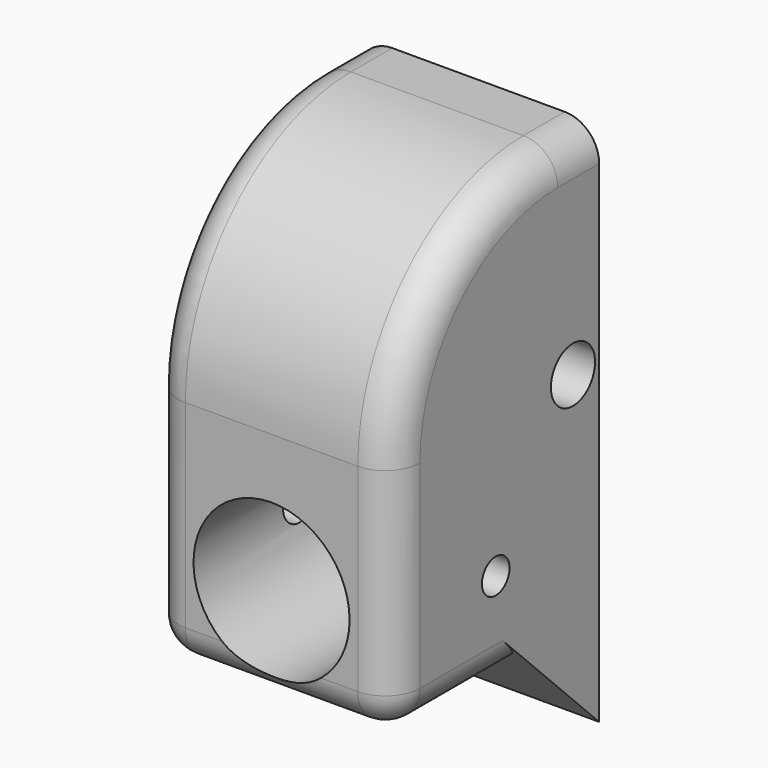
from build123d import *

# Parameters (mm, degrees)
F0_W         = 14
F0_H         = 30.5
F0_R         = 4.525
F1_DEPTH     = 15
F3_DEPTH     = 14.001
F4_R         = 1.6
F4_R_2       = 1
F5_DEPTH     = 14.001
F6_R         = 12
F7_T1_DEPTH  = 10
F7_T3_DEPTH  = 11.5
F7_T5_DEPTH  = 8
F7_S9_W      = 2
F7_S9_H      = 2
F7_T10_DEPTH = 2
F7_S15_W     = 2
F7_S15_H     = 2
F7_T16_DEPTH = 2
F7_T22_DEPTH = 13
F7_T25_ANGLE = 90
F7_T29_DEPTH = 13
F7_T32_ANGLE = 90


# Not quite as in the source:
# - a fillet or chamfer that OpenCascade refuses, or shapes differently, is made with other operations: its cross-section is extruded or revolved along the edge and cut away or added


with BuildPart() as f1:
    # F0 (on Front) → F1 (new body)
    with BuildSketch(Plane.XZ):
        with Locations((0, 4.75)):
            Rectangle(F0_W, F0_H)
        Circle(F0_R, mode=Mode.SUBTRACT)
    extrude(amount=F1_DEPTH)

    # F2 (on face) → F3 (cut, through all)
    with BuildSketch(Plane.YZ.offset(7)):
        Polygon((-15, -10.5), (0, -10.5), (-5, -5.5), (-15, -5.5), align=None)
    extrude(amount=-F3_DEPTH, mode=Mode.SUBTRACT)

    # F4 (on face) → F5 (cut, through all)
    with BuildSketch(Plane.YZ.offset(7)):
        with Locations((-1.9, 8)):
            Circle(F4_R)
        with Locations((-7.5, 0)):
            Circle(F4_R_2)
    extrude(amount=-F5_DEPTH, mode=Mode.SUBTRACT)

    # F6
    f6_edges = [f1.edges().sort_by_distance(p)[0] for p in [
        (0, -15, 20),
    ]]
    fillet(f6_edges, radius=F6_R)

    # F7: fillet of radius 2 on 9 edges, made by hand

    # F7_s2 → F7_t1 (cut)
    with BuildSketch(Plane.YZ.offset(-5)):
        with BuildLine():
            ThreePointArc((-15, -3.5), (-14.4142135624, -4.9142135624), (-13, -5.5))
            Line((-13, -5.5), (-15, -5.5))
            Line((-15, -5.5), (-15, -3.5))
        make_face()
    extrude(amount=F7_T1_DEPTH, mode=Mode.SUBTRACT)

    # F7_s4 → F7_t3 (cut)
    with BuildSketch(Plane.XY.offset(-3.5)):
        with BuildLine():
            ThreePointArc((7, -13), (6.4142135624, -14.4142135624), (5, -15))
            Line((5, -15), (7, -15))
            Line((7, -15), (7, -13))
        make_face()
        with BuildLine():
            ThreePointArc((-7, -13), (-6.4142135624, -14.4142135624), (-5, -15))
            Line((-5, -15), (-7, -15))
            Line((-7, -15), (-7, -13))
        make_face()
    extrude(amount=F7_T3_DEPTH, mode=Mode.SUBTRACT)

    # F7_s6 → F7_t5 (cut)
    with BuildSketch(Plane.XZ.offset(-5)):
        with BuildLine():
            ThreePointArc((5, 20), (6.4142135624, 19.4142135624), (7, 18))
            Line((7, 18), (7, 20))
            Line((7, 20), (5, 20))
        make_face()
        with BuildLine():
            ThreePointArc((-5, 20), (-6.4142135624, 19.4142135624), (-7, 18))
            Line((-7, 18), (-7, 20))
            Line((-7, 20), (-5, 20))
        make_face()
    extrude(amount=F7_T5_DEPTH, mode=Mode.SUBTRACT)


with BuildPart() as f7_tool8:
    # F7_s9 → F7_t10 (new body)
    with BuildSketch(Plane.YZ.offset(5)):
        with Locations((-14, -4.5)):
            Rectangle(F7_S9_W, F7_S9_H)
    extrude(amount=F7_T10_DEPTH)

    # F7_s11 → F7_t12 (revolve, cut)
    with BuildSketch(Plane(origin=(5, -13, -3.5), x_dir=(0, 0.7071067812, 0.7071067812), z_dir=(0, 0.7071067812, -0.7071067812))):
        with BuildLine():
            ThreePointArc((0, -2), (2, 0), (0, 2))
            Line((0, 2), (0, -2))
        make_face()
    revolve(axis=Axis((5, -13, -3.5), (1, 0, 0)), mode=Mode.SUBTRACT)


with BuildPart() as f1_1:
    add(f1.part)

    # F7_t7: cut F7_tool8
    add(f7_tool8.part, mode=Mode.SUBTRACT)


with BuildPart() as f7_tool14:
    # F7_s15 → F7_t16 (new body)
    with BuildSketch(Plane.YZ.offset(-5)):
        with Locations((-14, -4.5)):
            Rectangle(F7_S15_W, F7_S15_H)
    extrude(amount=-F7_T16_DEPTH)

    # F7_s17 → F7_t18 (revolve, cut)
    with BuildSketch(Plane(origin=(-5, -13, -3.5), x_dir=(0, 0.7071067812, 0.7071067812), z_dir=(0, -0.7071067812, 0.7071067812))):
        with BuildLine():
            ThreePointArc((0, -2), (2, 0), (0, 2))
            Line((0, 2), (0, -2))
        make_face()
    revolve(axis=Axis((-5, -13, -3.5), (-1, 0, 0)), mode=Mode.SUBTRACT)


with BuildPart() as f1_2:
    add(f1_1.part)

    # F7_t13: cut F7_tool14
    add(f7_tool14.part, mode=Mode.SUBTRACT)


with BuildPart() as f7_tool20:
    # F7_s21 → F7_t22 (new body)
    with BuildSketch(Plane.XZ):
        with BuildLine():
            ThreePointArc((-7, -3.5), (-6.4142135624, -4.9142135624), (-5, -5.5))
            Line((-5, -5.5), (-7, -5.5))
            Line((-7, -5.5), (-7, -3.5))
        make_face()
    extrude(amount=F7_T22_DEPTH)

    split(bisect_by=Plane(origin=(0, -5.25, -5.25), x_dir=(1, 0, 0), z_dir=(0, -0.7071067812, -0.7071067812)), keep=Keep.TOP)


with BuildPart() as f1_3:
    add(f1_2.part)

    # F7_t19: cut F7_tool20
    add(f7_tool20.part, mode=Mode.SUBTRACT)

    # F7_s24 → F7_t25 (revolve, cut)
    with BuildSketch(Plane.XZ.offset(3)):
        with BuildLine():
            ThreePointArc((-5, 20), (-6.4142135624, 19.4142135624), (-7, 18))
            Line((-7, 18), (-7, 20))
            Line((-7, 20), (-5, 20))
        make_face()
    revolve(axis=Axis((-7, -3, 8), (1, 0, 0)), revolution_arc=F7_T25_ANGLE, mode=Mode.SUBTRACT)


with BuildPart() as f7_tool27:
    # F7_s28 → F7_t29 (new body)
    with BuildSketch(Plane.XZ):
        with BuildLine():
            ThreePointArc((7, -3.5), (6.4142135624, -4.9142135624), (5, -5.5))
            Line((5, -5.5), (7, -5.5))
            Line((7, -5.5), (7, -3.5))
        make_face()
    extrude(amount=F7_T29_DEPTH)

    split(bisect_by=Plane(origin=(0, -5.25, -5.25), x_dir=(1, 0, 0), z_dir=(0, -0.7071067812, -0.7071067812)), keep=Keep.TOP)


with BuildPart() as f1_4:
    add(f1_3.part)

    # F7_t26: cut F7_tool27
    add(f7_tool27.part, mode=Mode.SUBTRACT)

    # F7_s31 → F7_t32 (revolve, cut)
    with BuildSketch(Plane.XZ.offset(3)):
        with BuildLine():
            ThreePointArc((7, 18), (6.4142135624, 19.4142135624), (5, 20))
            Line((5, 20), (7, 20))
            Line((7, 20), (7, 18))
        make_face()
    revolve(axis=Axis((7, -3, 8), (1, 0, 0)), revolution_arc=F7_T32_ANGLE, mode=Mode.SUBTRACT)


solid = f1_4.part
